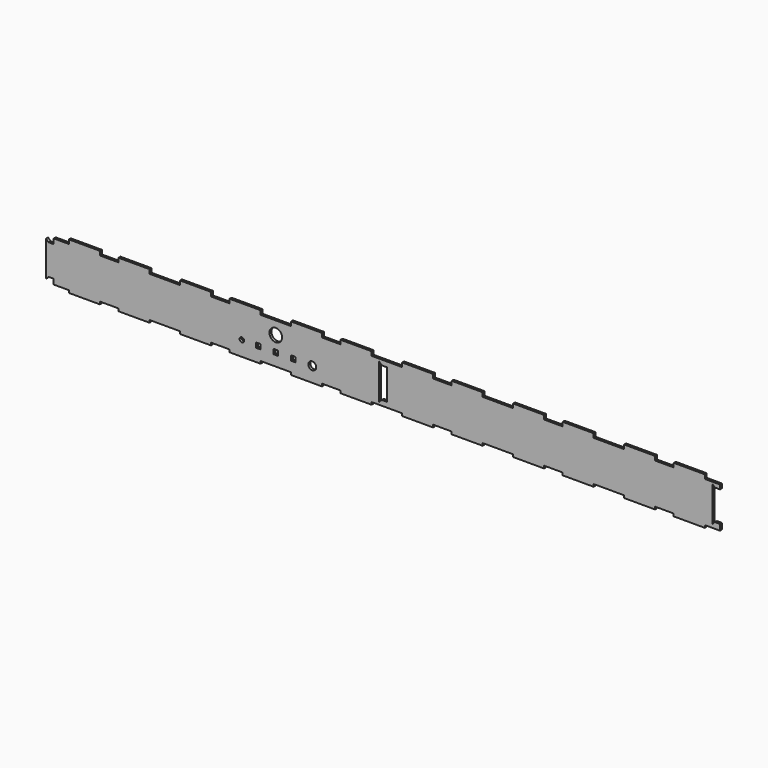
from build123d import *

# Parameters (mm, degrees)
F0_W      = 834.7400754492
F0_H      = 50.8
F1_DEPTH  = 3.048
F3_W      = 57.9247
F3_H      = 5.08
F3_W_2    = 115.8494
F3_H_2    = 3.1496
F4_DEPTH  = 3.048
F6_DEPTH  = 3.048
F7_DEPTH  = 3.049
F9_W      = 6.096
F9_H      = 6.096
F9_R      = 2.8702
F9_R_2    = 4.953
F9_R_3    = 7.9375
F10_DEPTH = 3.049
F11_DEPTH = 25.4
F12_W     = 38.1
F12_H     = 3.048
F12_H_2   = 5.08
F13_DEPTH = 3.048


# Not quite as in the source:
# - a feature names something its author has since deleted; it is built from what else it names


with BuildPart() as f1:
    # F0 (on Front) → F1 (new body)
    with BuildSketch(Plane.XZ):
        with Locations((417.3700377246, 25.4)):
            Rectangle(F0_W, F0_H)
    extrude(amount=F1_DEPTH)

    # F3 (on face) → F4 (join)
    with BuildSketch(Plane.XZ.offset(3.048)):
        with Locations((28.96235, 53.34)):
            Rectangle(F3_W, F3_H)
        with Locations((139.1233459082, 53.34)):
            Rectangle(F3_W_2, F3_H)
        with Locations((278.2466918164, 53.34)):
            Rectangle(F3_W_2, F3_H)
        with Locations((417.3700377246, 53.34)):
            Rectangle(F3_W_2, F3_H)
        with Locations((556.4933836328, 53.34)):
            Rectangle(F3_W_2, F3_H)
        with Locations((695.616729541, 53.34)):
            Rectangle(F3_W_2, F3_H)
        with Locations((805.7777254492, 53.34)):
            Rectangle(F3_W, F3_H)
        with Locations((28.96235, -1.5748)):
            Rectangle(F3_W, F3_H_2)
        with Locations((139.1233459082, -1.5748)):
            Rectangle(F3_W_2, F3_H_2)
        with Locations((278.2466918164, -1.5748)):
            Rectangle(F3_W_2, F3_H_2)
        with Locations((417.3700377246, -1.5748)):
            Rectangle(F3_W_2, F3_H_2)
        with Locations((556.4933836328, -1.5748)):
            Rectangle(F3_W_2, F3_H_2)
        with Locations((695.616729541, -1.5748)):
            Rectangle(F3_W_2, F3_H_2)
        with Locations((805.7777254492, -1.5748)):
            Rectangle(F3_W, F3_H_2)
    extrude(amount=-F4_DEPTH)

    # F5 (on face) → F6 (join)
    with BuildSketch(Plane.XZ.offset(3.048)):
        Polygon((-6.35, 6.35), (0, 6.35), (0, 44.45), (-6.35, 44.45), (-9.525, 47.625), (-9.525, 3.175), align=None)
    extrude(amount=-F6_DEPTH)

    # F5 (on face) → F7 (cut, through all)
    with BuildSketch(Plane.XZ.offset(3.048)):
        Polygon((828.3900754492, 7.3152), (834.7400754492, 7.3152), (834.7400754492, 45.4152), (828.3900754492, 45.4152), (825.2150754492, 48.5902), (825.2150754492, 4.1402), align=None)
    extrude(amount=-F7_DEPTH, mode=Mode.SUBTRACT)

    # F9 (on face) → F10 (cut, through all)
    with BuildSketch(Plane.XZ.offset(3.048)):
        with Locations((256.3264918164, 15.621)):
            Rectangle(F9_W, F9_H)
        with Locations((278.2466918164, 15.621)):
            Rectangle(F9_W, F9_H)
        with Locations((300.1668918164, 15.621)):
            Rectangle(F9_W, F9_H)
        with Locations((235.7016918164, 15.621)):
            Circle(F9_R)
        with Locations((323.9666918164, 15.621)):
            Circle(F9_R_2)
        with Locations((278.2466918164, 34.671)):
            Circle(F9_R_3)
    extrude(amount=-F10_DEPTH, mode=Mode.SUBTRACT)

    # F8 (on face) → F11 (cut)
    with BuildSketch(Plane.XZ.offset(3.048)):
        Polygon((411.0200377246, 6.35), (417.3700377246, 6.35), (417.3700377246, 44.45), (411.0200377246, 44.45), (407.8450377246, 47.625), (407.8450377246, 3.175), align=None)
    extrude(amount=-F11_DEPTH, mode=Mode.SUBTRACT)

    # F12 (on face) → F13 (cut, through all)
    with BuildSketch(Plane.XZ.offset(3.048)):
        with Locations((139.1233459082, -1.6256)):
            Rectangle(F12_W, F12_H)
        with Locations((278.2466918164, -1.6256)):
            Rectangle(F12_W, F12_H)
        with Locations((417.3700377246, -1.6256)):
            Rectangle(F12_W, F12_H)
        with Locations((556.4933836328, -1.6256)):
            Rectangle(F12_W, F12_H)
        with Locations((695.616729541, -1.6256)):
            Rectangle(F12_W, F12_H)
        with Locations((834.7400754492, -1.6256)):
            Rectangle(F12_W, F12_H)
        with Locations((0, -1.6256)):
            Rectangle(F12_W, F12_H)
        with Locations((0, 53.34)):
            Rectangle(F12_W, F12_H_2)
        with Locations((139.1233459082, 53.34)):
            Rectangle(F12_W, F12_H_2)
        with Locations((278.2466918164, 53.34)):
            Rectangle(F12_W, F12_H_2)
        with Locations((417.3700377246, 53.34)):
            Rectangle(F12_W, F12_H_2)
        with Locations((556.4933836328, 53.34)):
            Rectangle(F12_W, F12_H_2)
        with Locations((695.616729541, 53.34)):
            Rectangle(F12_W, F12_H_2)
        with Locations((834.7400754492, 53.34)):
            Rectangle(F12_W, F12_H_2)
    extrude(amount=-F13_DEPTH, mode=Mode.SUBTRACT)


solid = f1.part
